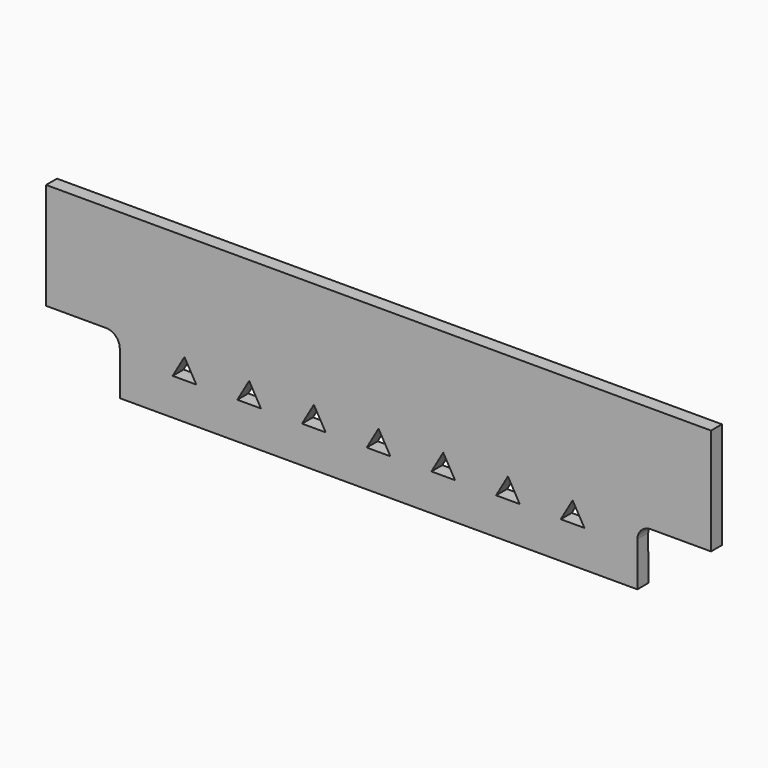
from build123d import *

# Parameters (mm, degrees)
F1_DEPTH = 25


# Not quite as in the source:
# - a feature names something its author has since deleted; it is built from what else it names


with BuildPart() as f1:
    # F0 (on Front) → F1 (new body)
    with BuildSketch(Plane.XZ):
        with BuildLine():
            Line((609, -45), (609, 150))
            Line((609, 150), (-609, 150))
            Line((-609, 150), (-609, -45))
            Line((-609, -45), (-499, -45))
            ThreePointArc((-499, -45), (-481.3223304703, -52.3223304703), (-474, -70))
            Line((-474, -70), (-474, -150))
            Line((-474, -150), (474.1005301476, -150))
            Line((474.1005301476, -150), (474.0229112381, -68.9299359934))
            ThreePointArc((474.0229112381, -68.9299359934), (481.7047925737, -51.947969641), (499, -45))
            Line((499, -45), (609, -45))
        make_face()
        Polygon((-377.1515345675, -82.4994803672), (-355.4999994674, -45), (-333.8502643907, -82.5005196112), align=None, mode=Mode.SUBTRACT)
        Polygon((-258.6515341126, -82.4994803672), (-236.9999990125, -45), (-215.3502639358, -82.5005196112), align=None, mode=Mode.SUBTRACT)
        Polygon((-140.1515340625, -82.4994803672), (-118.4999989624, -45), (-96.8502638857, -82.5005196112), align=None, mode=Mode.SUBTRACT)
        Polygon((-21.651534291, -82.4994803674), (8.087e-07, -45), (21.6497358858, -82.500519611), align=None, mode=Mode.SUBTRACT)
        Polygon((96.8493649054, -82.5), (118.5, -45), (140.1506350946, -82.5), align=None, mode=Mode.SUBTRACT)
        Polygon((215.3493649054, -82.5), (237, -45), (258.6506350946, -82.5), align=None, mode=Mode.SUBTRACT)
        Polygon((333.8493649054, -82.5), (355.5, -45), (377.1506350946, -82.5), align=None, mode=Mode.SUBTRACT)
    extrude(amount=F1_DEPTH)


solid = f1.part
